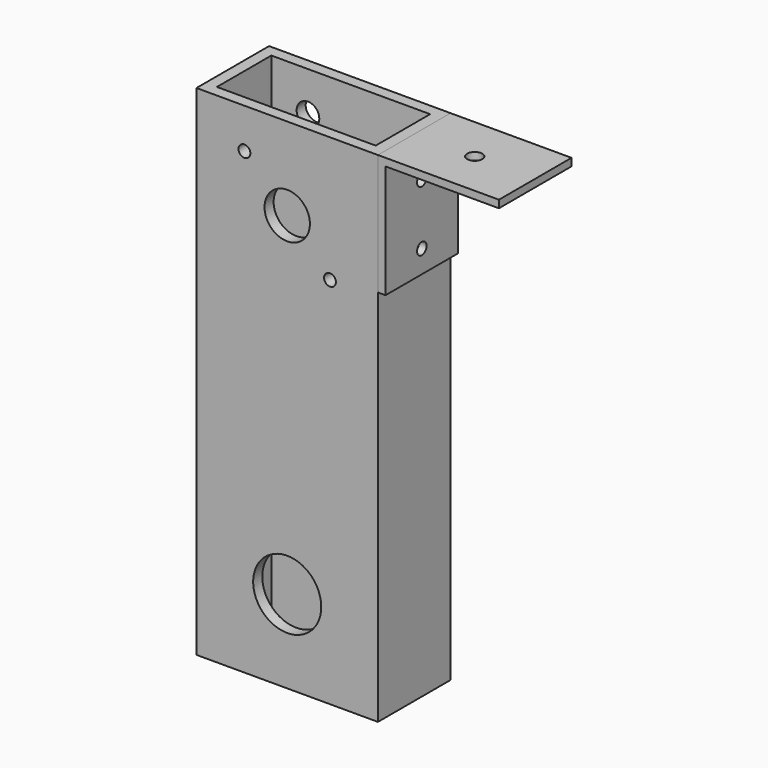
from build123d import *

# Parameters (mm, degrees)
F0_W          = 76.2
F0_H          = 38.1
F1_DEPTH      = 104.775
F2_T          = -4.7625
F3_R          = 9.525
F3_R_2        = 2.4892
F3_R_3        = 14.2875
F4_DEPTH      = 19.051
F3_R_4        = 4.7625
F5_DEPTH      = 25.4
F7_DEPTH      = 19.05
F8_R          = 2.0193
F9_DEPTH      = 38.101
F9_DEPTH_BACK = 88.901
F10_R         = 3.175
F11_DEPTH     = 209.551
F8_R_2        = 2.4892
F12_DEPTH     = 88.901


with BuildPart() as f1:
    # F0 (on Top) → F1 (new body, symmetric)
    with BuildSketch(Plane.XY):
        Rectangle(F0_W, F0_H)
    extrude(amount=F1_DEPTH, both=True)

    # F2
    f2_openings = [f1.faces().sort_by_distance(p)[0] for p in [
        (0, 0, 104.775),
        (0, 0, -104.775),
    ]]
    offset(amount=F2_T, openings=f2_openings)

    # F3 (on Front) → F4 (cut, through all)
    with BuildSketch(Plane.XZ):
        with Locations((0, 70.01256)):
            Circle(F3_R)
        with Locations((-17.9605122421, 87.9730722421)):
            Circle(F3_R_2)
        with Locations((17.9605122421, 52.0520477579)):
            Circle(F3_R_2)
        with Locations((0, -70.01256)):
            Circle(F3_R_3)
    extrude(amount=F4_DEPTH, mode=Mode.SUBTRACT)

    # F3 (on Front) → F5 (cut)
    with BuildSketch(Plane.XZ):
        with Locations((0, 70.01256)):
            Circle(F3_R_3)
        with Locations((0, 70.01256)):
            Circle(F3_R, mode=Mode.SUBTRACT)
        with Locations((0, -70.01256)):
            Circle(F3_R_3)
        with Locations((0, 70.01256)):
            Circle(F3_R)
        with Locations((-17.9605122421, 87.9730722421)):
            Circle(F3_R_4)
        with Locations((-17.9605122421, 87.9730722421)):
            Circle(F3_R_2, mode=Mode.SUBTRACT)
        with Locations((17.9605122421, 52.0520477579)):
            Circle(F3_R_4)
        with Locations((17.9605122421, 52.0520477579)):
            Circle(F3_R_2, mode=Mode.SUBTRACT)
        with Locations((-17.9605122421, 87.9730722421)):
            Circle(F3_R_2)
        with Locations((17.9605122421, 52.0520477579)):
            Circle(F3_R_2)
    extrude(amount=-F5_DEPTH, mode=Mode.SUBTRACT)


with BuildPart() as f7:
    # F6 (on Front) → F7 (new body, symmetric)
    with BuildSketch(Plane.XZ):
        Polygon((38.1, 104.775), (38.1, 53.975), (41.275, 53.975), (41.275, 101.6), (88.9, 101.6), (88.9, 104.775), align=None)
    extrude(amount=F7_DEPTH, both=True)


with BuildPart() as f9_tool:
    # F8 (on Right) → F9 (new body, two sides)
    with BuildSketch(Plane.YZ) as f9_sk:
        with Locations((0, 88.9)):
            Circle(F8_R)
        with Locations((0, 63.5)):
            Circle(F8_R)
    extrude(amount=-F9_DEPTH)
    extrude(f9_sk.sketch, amount=F9_DEPTH_BACK)


with BuildPart() as f1_1:
    add(f1.part)

    # F9: cut by f9_tool
    add(f9_tool.part, mode=Mode.SUBTRACT)


with BuildPart() as f7_1:
    add(f7.part)

    # F9: cut by f9_tool
    add(f9_tool.part, mode=Mode.SUBTRACT)

    # F10 (on face) → F11 (cut, through all)
    with BuildSketch(Plane.XY.offset(104.775)):
        with Locations((63.5, 0)):
            Circle(F10_R)
    extrude(amount=-F11_DEPTH, mode=Mode.SUBTRACT)

    # F8 (on Right) → F12 (cut, through all)
    with BuildSketch(Plane.YZ):
        with Locations((0, 88.9)):
            Circle(F8_R_2)
        with Locations((0, 88.9)):
            Circle(F8_R, mode=Mode.SUBTRACT)
        with Locations((0, 63.5)):
            Circle(F8_R_2)
        with Locations((0, 63.5)):
            Circle(F8_R, mode=Mode.SUBTRACT)
        with Locations((0, 88.9)):
            Circle(F8_R)
        with Locations((0, 63.5)):
            Circle(F8_R)
    extrude(amount=F12_DEPTH, mode=Mode.SUBTRACT)


solid = Compound([f1_1.part, f7_1.part])
